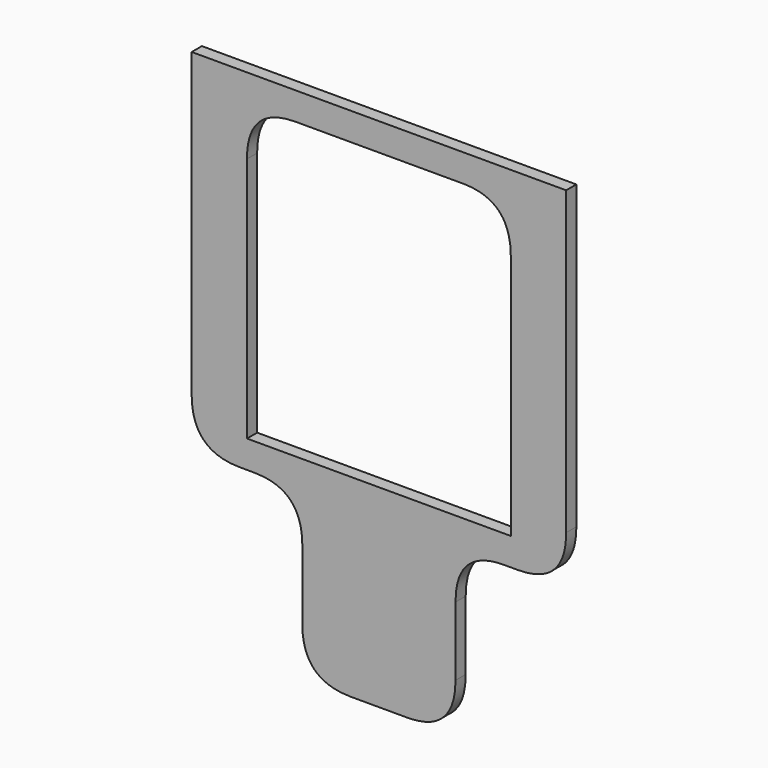
from build123d import *

# Parameters (mm, degrees)
F1_DEPTH    = 20
F2_T1_DEPTH = 20
F2_T3_DEPTH = 401
F3_W        = 414
F3_H        = 462.4
F4_DEPTH    = 25.4
F5_T1_DEPTH = 20


# Not quite as in the source:
# - a fillet or chamfer that OpenCascade refuses, or shapes differently, is made with other operations: its cross-section is extruded or revolved along the edge and cut away or added


with BuildPart() as f1:
    # F0 (on Front) → F1 (new body)
    with BuildSketch(Plane.XZ):
        Polygon((293.8, 477), (-293.8, 477), (-293.8, -72.2), (-120.2, -72.2), (-120.2, -332.6), (120.2, -332.6), (120.2, -72.2), (293.8, -72.2), align=None)
    extrude(amount=F1_DEPTH)

    # F2: fillet of radius 76.2 on 6 edges, made by hand

    # F2_s2 → F2_t1 (join)
    with BuildSketch(Plane.XZ):
        with BuildLine():
            add(Edge.make_bspline(
                [(-196.4, -72.2), (-120.2, -72.2), (-120.2, -148.4)],
                knots=[0, 0, 0, 1, 1, 1], degree=2, weights=[1, 1, 1]))
            Line((-120.2, -148.4), (-120.2, -72.2))
            Line((-120.2, -72.2), (-196.4, -72.2))
        make_face()
        with BuildLine():
            add(Edge.make_bspline(
                [(120.2, -148.4), (120.2, -72.2), (196.4, -72.2)],
                knots=[0, 0, 0, 1, 1, 1], degree=2, weights=[1, 1, 1]))
            Line((196.4, -72.2), (120.2, -72.2))
            Line((120.2, -72.2), (120.2, -148.4))
        make_face()
    extrude(amount=F2_T1_DEPTH)

    # F2_s4 → F2_t3 (cut)
    with BuildSketch(Plane.XZ.offset(-190.5)):
        with BuildLine():
            add(Edge.make_bspline(
                [(-293.8, 4), (-293.8, -72.2), (-217.6, -72.2)],
                knots=[0, 0, 0, 1, 1, 1], degree=2, weights=[1, 1, 1]))
            Line((-217.6, -72.2), (-293.8, -72.2))
            Line((-293.8, -72.2), (-293.8, 4))
        make_face()
        with BuildLine():
            add(Edge.make_bspline(
                [(44, -332.6), (120.2, -332.6), (120.2, -256.4)],
                knots=[0, 0, 0, 1, 1, 1], degree=2, weights=[1, 1, 1]))
            Line((120.2, -256.4), (120.2, -332.6))
            Line((120.2, -332.6), (44, -332.6))
        make_face()
        with BuildLine():
            add(Edge.make_bspline(
                [(293.8, 4), (293.8, -72.2), (217.6, -72.2)],
                knots=[0, 0, 0, 1, 1, 1], degree=2, weights=[1, 1, 1]))
            Line((217.6, -72.2), (293.8, -72.2))
            Line((293.8, -72.2), (293.8, 4))
        make_face()
        with BuildLine():
            add(Edge.make_bspline(
                [(-120.2, -256.4), (-120.2, -332.6), (-44, -332.6)],
                knots=[0, 0, 0, 1, 1, 1], degree=2, weights=[1, 1, 1]))
            Line((-44, -332.6), (-120.2, -332.6))
            Line((-120.2, -332.6), (-120.2, -256.4))
        make_face()
    extrude(amount=F2_T3_DEPTH, mode=Mode.SUBTRACT)

    # F3 (on Front) → F4 (cut)
    with BuildSketch(Plane.XZ):
        with Locations((0, 202.4)):
            Rectangle(F3_W, F3_H)
    extrude(amount=F4_DEPTH, mode=Mode.SUBTRACT)

    # F5: fillet of radius 76.2 on 2 edges, made by hand

    # F5_s2 → F5_t1 (join)
    with BuildSketch(Plane.XZ):
        with BuildLine():
            add(Edge.make_bspline(
                [(-130.8, 433.6), (-207, 433.6), (-207, 357.4)],
                knots=[0, 0, 0, 1, 1, 1], degree=2, weights=[1, 1, 1]))
            Line((-207, 357.4), (-207, 433.6))
            Line((-207, 433.6), (-130.8, 433.6))
        make_face()
        with BuildLine():
            add(Edge.make_bspline(
                [(207, 357.4), (207, 433.6), (130.8, 433.6)],
                knots=[0, 0, 0, 1, 1, 1], degree=2, weights=[1, 1, 1]))
            Line((130.8, 433.6), (207, 433.6))
            Line((207, 433.6), (207, 357.4))
        make_face()
    extrude(amount=F5_T1_DEPTH)


solid = f1.part
